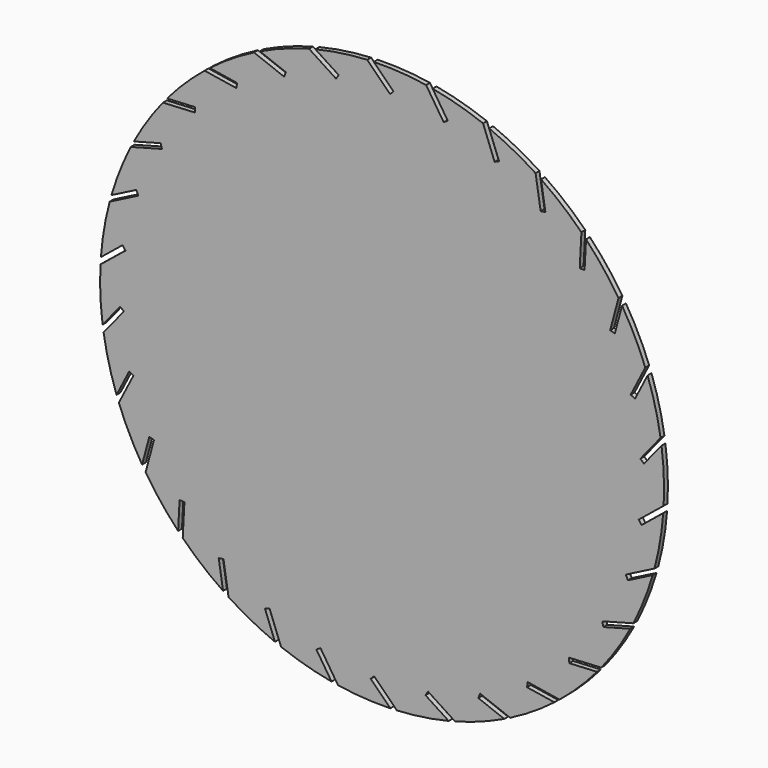
from build123d import *

# Parameters (mm, degrees)
F0_R            = 175
F1_DEPTH        = 3
F3_DEPTH        = 3.001
F3_COPIES_COUNT = 30


# Not quite as in the source:
# - a pattern or mirror of a feature is missing from the dataset's text; its kind, count and spacing are read off the source's solid


with BuildPart() as f1:
    # F0 (on Front) → F1 (new body)
    with BuildSketch(Plane.XZ):
        Circle(F0_R)
    extrude(amount=-F1_DEPTH)

    # F2 (on face) → F3 (cut, through all)
    with BuildSketch(Plane.XZ):
        with BuildLine():
            ThreePointArc((-5.1165300167, 174.9251872104), (-7.1549450675, 174.8536724266), (-9.1923881554, 174.758404662))
            Line((-9.1923881554, 174.758404662), (4.9497474683, 160.6162690382))
            Line((4.9497474683, 160.6162690382), (7.0710678119, 162.7375893818))
            Line((7.0710678119, 162.7375893818), (-5.1165300167, 174.9251872104))
        make_face()
    f3 = extrude(amount=-F3_DEPTH, mode=Mode.SUBTRACT)

    # F3_copies: F3 ×30 about axis
    f3_copies_axis = Axis((0, 0, 0), (0, 1, 0))
    for i in range(1, F3_COPIES_COUNT):
        add(f3.rotate(f3_copies_axis, i * 360 / F3_COPIES_COUNT), mode=Mode.SUBTRACT)


solid = f1.part
